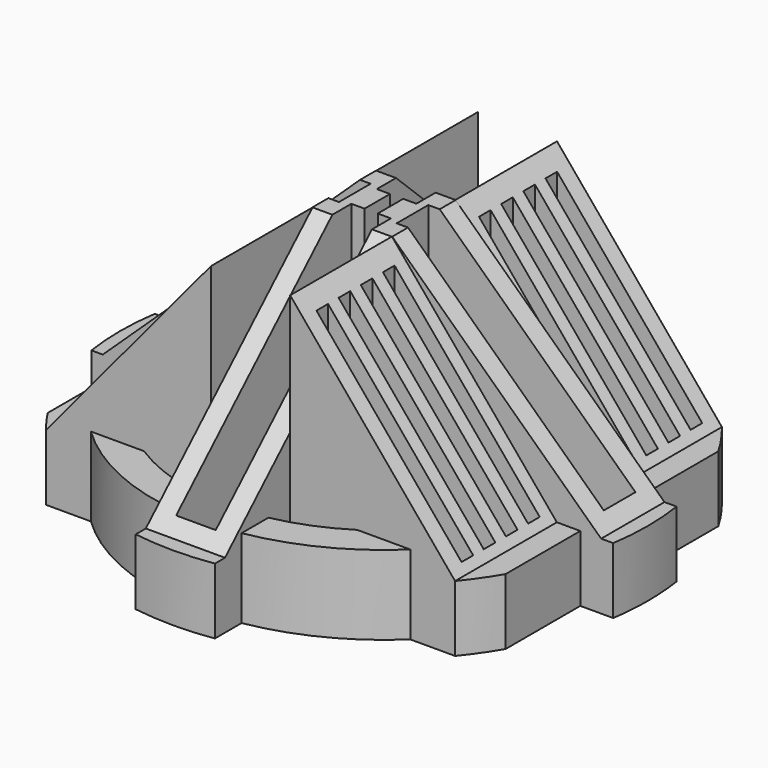
from build123d import *

# Parameters (mm, degrees)
F2_DEPTH  = 12.7
F3_DEPTH  = 25.4
F4_DEPTH  = 38.1
F5_DEPTH  = 50.8
F6_DEPTH  = 50.8
F7_DEPTH  = 50.8
F11_DEPTH = 15.24
F12_DEPTH = 15.24
F13_DEPTH = 15.24
F15_DEPTH = 15.24
F16_W     = 39.878
F16_H     = 7.62
F16_W_2   = 7.62
F16_H_2   = 42.164
F17_DEPTH = 46.99
F18_DEPTH = 50.8
F21_DEPTH = 24.4856
F19_W     = 27.94
F19_H     = 2.794
F22_DEPTH = 46.99
F24_DEPTH = 24.4856
F26_DEPTH = 24.4856
F28_DEPTH = 24.4856
F29_DEPTH = 50.801
F30_DEPTH = 25.4
F31_DEPTH = 10.16
F33_DEPTH = 25.4
F35_DEPTH = 46.99


# Not quite as in the source:
# - after a boolean that leaves OpenCascade's solid faulty, fix() repairs it
# - a feature names something its author has since deleted; it is built from what else it names


with BuildPart() as f2:
    # F1 (on Top) → F2 (new body)
    with BuildSketch(Plane.XY):
        with BuildLine():
            ThreePointArc((50.2252486305, -7.62), (50.6561083702, -3.8208225272), (50.8, 0))
            ThreePointArc((50.8, 0), (50.6561083702, 3.8208225272), (50.2252486305, 7.62))
            Line((50.2252486305, 7.62), (43.8856464383, 7.62))
            Line((43.8856464383, 7.62), (43.8856464383, -7.62))
            Line((43.8856464383, -7.62), (50.2252486305, -7.62))
        make_face()
        with BuildLine():
            Line((43.8856464383, 7.62), (50.2252486305, 7.62))
            ThreePointArc((50.2252486305, 7.62), (48.8754001329, 13.850460709), (46.7558464383, 19.8628))
            Line((46.7558464383, 19.8628), (43.8856464383, 19.8628))
            Line((43.8856464383, 19.8628), (43.8856464383, 7.62))
        make_face()
        with BuildLine():
            ThreePointArc((46.7558464383, -19.8628), (48.8754001329, -13.850460709), (50.2252486305, -7.62))
            Line((50.2252486305, -7.62), (43.8856464383, -7.62))
            Line((43.8856464383, -7.62), (43.8856464383, -19.8628))
            Line((43.8856464383, -19.8628), (46.7558464383, -19.8628))
        make_face()
        with BuildLine():
            Line((43.8856464383, 19.8628), (46.7558464383, 19.8628))
            ThreePointArc((46.7558464383, 19.8628), (43.4950311771, 26.2454236564), (39.3683940318, 32.1056))
            Line((39.3683940318, 32.1056), (30.7413882029, 32.1056))
            ThreePointArc((30.7413882029, 32.1056), (35.7808122406, 26.3730160468), (39.7652068542, 19.8628))
            Line((39.7652068542, 19.8628), (43.8856464383, 19.8628))
        make_face()
        with BuildLine():
            ThreePointArc((39.3683940318, -32.1056), (43.4950311771, -26.2454236564), (46.7558464383, -19.8628))
            Line((46.7558464383, -19.8628), (43.8856464383, -19.8628))
            Line((43.8856464383, -19.8628), (39.7652068542, -19.8628))
            ThreePointArc((39.7652068542, -19.8628), (35.7808122406, -26.3730160468), (30.7413882029, -32.1056))
            Line((30.7413882029, -32.1056), (39.3683940318, -32.1056))
        make_face()
        with BuildLine():
            Line((30.7413882029, 32.1056), (39.3683940318, 32.1056))
            ThreePointArc((39.3683940318, 32.1056), (25.1805025773, 44.1200894146), (7.62, 50.2252486305))
            Line((7.62, 50.2252486305), (7.62, 43.7919867099))
            ThreePointArc((7.62, 43.7919867099), (20.0509833873, 39.670651182), (30.7413882029, 32.1056))
        make_face()
        with BuildLine():
            ThreePointArc((7.62, -50.2252486305), (25.1805025773, -44.1200894146), (39.3683940318, -32.1056))
            Line((39.3683940318, -32.1056), (30.7413882029, -32.1056))
            ThreePointArc((30.7413882029, -32.1056), (20.0509833873, -39.670651182), (7.62, -43.7919867099))
            Line((7.62, -43.7919867099), (7.62, -50.2252486305))
        make_face()
        with BuildLine():
            Line((7.62, 43.7919867099), (7.62, 50.2252486305))
            ThreePointArc((7.62, 50.2252486305), (0, 50.8), (-7.62, 50.2252486305))
            Line((-7.62, 50.2252486305), (-7.62, 43.7919867099))
            ThreePointArc((-7.62, 43.7919867099), (0, 44.45), (7.62, 43.7919867099))
        make_face()
        with BuildLine():
            Line((20.5143961315, 32.1056), (30.7413882029, 32.1056))
            ThreePointArc((30.7413882029, 32.1056), (20.0509833873, 39.670651182), (7.62, 43.7919867099))
            Line((7.62, 43.7919867099), (7.62, 37.33022368))
            ThreePointArc((7.62, 37.33022368), (14.3076984372, 35.3114679025), (20.5143961315, 32.1056))
        make_face()
        with BuildLine():
            ThreePointArc((-7.62, -50.2252486305), (0, -50.8), (7.62, -50.2252486305))
            Line((7.62, -50.2252486305), (7.62, -43.7919867099))
            ThreePointArc((7.62, -43.7919867099), (0, -44.45), (-7.62, -43.7919867099))
            Line((-7.62, -43.7919867099), (-7.62, -50.2252486305))
        make_face()
        with BuildLine():
            ThreePointArc((7.62, -43.7919867099), (20.0509833873, -39.670651182), (30.7413882029, -32.1056))
            Line((30.7413882029, -32.1056), (20.5143961315, -32.1056))
            ThreePointArc((20.5143961315, -32.1056), (14.3076984372, -35.3114679025), (7.62, -37.33022368))
            Line((7.62, -37.33022368), (7.62, -43.7919867099))
        make_face()
        with BuildLine():
            Line((-7.62, 43.7919867099), (-7.62, 50.2252486305))
            ThreePointArc((-7.62, 50.2252486305), (-25.1805025773, 44.1200894146), (-39.3683940318, 32.1056))
            Line((-39.3683940318, 32.1056), (-30.7413882029, 32.1056))
            ThreePointArc((-30.7413882029, 32.1056), (-20.0509833873, 39.670651182), (-7.62, 43.7919867099))
        make_face()
        with BuildLine():
            ThreePointArc((-39.3683940318, -32.1056), (-25.1805025773, -44.1200894146), (-7.62, -50.2252486305))
            Line((-7.62, -50.2252486305), (-7.62, -43.7919867099))
            ThreePointArc((-7.62, -43.7919867099), (-20.0509833873, -39.670651182), (-30.7413882029, -32.1056))
            Line((-30.7413882029, -32.1056), (-39.3683940318, -32.1056))
        make_face()
        with BuildLine():
            Line((-30.7413882029, 32.1056), (-39.3683940318, 32.1056))
            ThreePointArc((-39.3683940318, 32.1056), (-43.4950311771, 26.2454236564), (-46.7558464383, 19.8628))
            Line((-46.7558464383, 19.8628), (-42.6407977939, 19.8628))
            Line((-42.6407977939, 19.8628), (-39.7652068542, 19.8628))
            ThreePointArc((-39.7652068542, 19.8628), (-35.7808122406, 26.3730160468), (-30.7413882029, 32.1056))
        make_face()
        with BuildLine():
            Line((-7.62, 37.33022368), (-7.62, 43.7919867099))
            ThreePointArc((-7.62, 43.7919867099), (-20.0509833873, 39.670651182), (-30.7413882029, 32.1056))
            Line((-30.7413882029, 32.1056), (-20.5143961315, 32.1056))
            ThreePointArc((-20.5143961315, 32.1056), (-14.3076984372, 35.3114679025), (-7.62, 37.33022368))
        make_face()
        with BuildLine():
            ThreePointArc((-46.7558464383, -19.8628), (-43.4950311771, -26.2454236564), (-39.3683940318, -32.1056))
            Line((-39.3683940318, -32.1056), (-30.7413882029, -32.1056))
            ThreePointArc((-30.7413882029, -32.1056), (-35.7808122406, -26.3730160468), (-39.7652068542, -19.8628))
            Line((-39.7652068542, -19.8628), (-42.6407977939, -19.8628))
            Line((-42.6407977939, -19.8628), (-46.7558464383, -19.8628))
        make_face()
        with BuildLine():
            ThreePointArc((-30.7413882029, -32.1056), (-20.0509833873, -39.670651182), (-7.62, -43.7919867099))
            Line((-7.62, -43.7919867099), (-7.62, -37.33022368))
            ThreePointArc((-7.62, -37.33022368), (-14.2009349705, -35.3545392554), (-20.32, -32.2289869527))
            ThreePointArc((-20.32, -32.2289869527), (-20.4172912734, -32.1674403249), (-20.5143961315, -32.1056))
            Line((-20.5143961315, -32.1056), (-30.7413882029, -32.1056))
        make_face()
        with BuildLine():
            Line((-42.6407977939, 19.8628), (-46.7558464383, 19.8628))
            ThreePointArc((-46.7558464383, 19.8628), (-48.8754001329, 13.850460709), (-50.2252486305, 7.62))
            Line((-50.2252486305, 7.62), (-42.6407977939, 7.62))
            Line((-42.6407977939, 7.62), (-42.6407977939, 19.8628))
        make_face()
        with BuildLine():
            ThreePointArc((-50.2252486305, -7.62), (-48.8754001329, -13.850460709), (-46.7558464383, -19.8628))
            Line((-46.7558464383, -19.8628), (-42.6407977939, -19.8628))
            Line((-42.6407977939, -19.8628), (-42.6407977939, -7.62))
            Line((-42.6407977939, -7.62), (-50.2252486305, -7.62))
        make_face()
        with BuildLine():
            Line((-42.6407977939, 7.62), (-50.2252486305, 7.62))
            ThreePointArc((-50.2252486305, 7.62), (-50.8, 0), (-50.2252486305, -7.62))
            Line((-50.2252486305, -7.62), (-42.6407977939, -7.62))
            Line((-42.6407977939, -7.62), (-42.6407977939, 7.62))
        make_face()
    extrude(amount=F2_DEPTH)

    # F1 (on Top) → F3 (join)
    with BuildSketch(Plane.XY):
        with BuildLine():
            ThreePointArc((-30.7413882029, -32.1056), (-20.0509833873, -39.670651182), (-7.62, -43.7919867099))
            Line((-7.62, -43.7919867099), (-7.62, -37.33022368))
            ThreePointArc((-7.62, -37.33022368), (-14.2009349705, -35.3545392554), (-20.32, -32.2289869527))
            ThreePointArc((-20.32, -32.2289869527), (-20.4172912734, -32.1674403249), (-20.5143961315, -32.1056))
            Line((-20.5143961315, -32.1056), (-30.7413882029, -32.1056))
        make_face()
        with BuildLine():
            ThreePointArc((7.62, -43.7919867099), (20.0509833873, -39.670651182), (30.7413882029, -32.1056))
            Line((30.7413882029, -32.1056), (20.5143961315, -32.1056))
            ThreePointArc((20.5143961315, -32.1056), (14.3076984372, -35.3114679025), (7.62, -37.33022368))
            Line((7.62, -37.33022368), (7.62, -43.7919867099))
        make_face()
        with BuildLine():
            Line((20.5143961315, -32.1056), (30.7413882029, -32.1056))
            ThreePointArc((30.7413882029, -32.1056), (35.7808122406, -26.3730160468), (39.7652068542, -19.8628))
            Line((39.7652068542, -19.8628), (32.5127540538, -19.8628))
            ThreePointArc((32.5127540538, -19.8628), (27.2110492659, -26.667748271), (20.5143961315, -32.1056))
        make_face()
        with BuildLine():
            Line((7.62, 37.33022368), (7.62, 43.7919867099))
            ThreePointArc((7.62, 43.7919867099), (0, 44.45), (-7.62, 43.7919867099))
            Line((-7.62, 43.7919867099), (-7.62, 37.33022368))
            ThreePointArc((-7.62, 37.33022368), (0, 38.1), (7.62, 37.33022368))
        make_face()
        with BuildLine():
            ThreePointArc((-7.62, -43.7919867099), (0, -44.45), (7.62, -43.7919867099))
            Line((7.62, -43.7919867099), (7.62, -37.33022368))
            ThreePointArc((7.62, -37.33022368), (0, -38.1), (-7.62, -37.33022368))
            Line((-7.62, -37.33022368), (-7.62, -43.7919867099))
        make_face()
        with BuildLine():
            Line((-37.33022368, 7.62), (-42.6407977939, 7.62))
            Line((-42.6407977939, 7.62), (-42.6407977939, -7.62))
            Line((-42.6407977939, -7.62), (-37.33022368, -7.62))
            ThreePointArc((-37.33022368, -7.62), (-38.1, 0), (-37.33022368, 7.62))
        make_face()
        with BuildLine():
            Line((-42.6407977939, -7.62), (-42.6407977939, -19.8628))
            Line((-42.6407977939, -19.8628), (-39.7652068542, -19.8628))
            Line((-39.7652068542, -19.8628), (-32.5127540538, -19.8628))
            ThreePointArc((-32.5127540538, -19.8628), (-35.4539408619, -13.9509167211), (-37.33022368, -7.62))
            Line((-37.33022368, -7.62), (-42.6407977939, -7.62))
        make_face()
        with BuildLine():
            ThreePointArc((-39.7652068542, -19.8628), (-35.7808122406, -26.3730160468), (-30.7413882029, -32.1056))
            Line((-30.7413882029, -32.1056), (-20.5143961315, -32.1056))
            ThreePointArc((-20.5143961315, -32.1056), (-27.2110492659, -26.667748271), (-32.5127540538, -19.8628))
            Line((-32.5127540538, -19.8628), (-39.7652068542, -19.8628))
        make_face()
        with BuildLine():
            Line((-39.7652068542, 19.8628), (-42.6407977939, 19.8628))
            Line((-42.6407977939, 19.8628), (-42.6407977939, 7.62))
            Line((-42.6407977939, 7.62), (-37.33022368, 7.62))
            ThreePointArc((-37.33022368, 7.62), (-35.4539408619, 13.9509167211), (-32.5127540538, 19.8628))
            Line((-32.5127540538, 19.8628), (-39.7652068542, 19.8628))
        make_face()
        with BuildLine():
            Line((-20.5143961315, 32.1056), (-30.7413882029, 32.1056))
            ThreePointArc((-30.7413882029, 32.1056), (-35.7808122406, 26.3730160468), (-39.7652068542, 19.8628))
            Line((-39.7652068542, 19.8628), (-32.5127540538, 19.8628))
            ThreePointArc((-32.5127540538, 19.8628), (-27.2110492659, 26.667748271), (-20.5143961315, 32.1056))
        make_face()
        with BuildLine():
            Line((-7.62, 37.33022368), (-7.62, 43.7919867099))
            ThreePointArc((-7.62, 43.7919867099), (-20.0509833873, 39.670651182), (-30.7413882029, 32.1056))
            Line((-30.7413882029, 32.1056), (-20.5143961315, 32.1056))
            ThreePointArc((-20.5143961315, 32.1056), (-14.3076984372, 35.3114679025), (-7.62, 37.33022368))
        make_face()
        with BuildLine():
            ThreePointArc((39.7652068542, 19.8628), (35.7808122406, 26.3730160468), (30.7413882029, 32.1056))
            Line((30.7413882029, 32.1056), (20.5143961315, 32.1056))
            ThreePointArc((20.5143961315, 32.1056), (27.2110492659, 26.667748271), (32.5127540538, 19.8628))
            Line((32.5127540538, 19.8628), (39.7652068542, 19.8628))
        make_face()
        with BuildLine():
            Line((37.33022368, 7.62), (43.8856464383, 7.62))
            Line((43.8856464383, 7.62), (43.8856464383, 19.8628))
            Line((43.8856464383, 19.8628), (39.7652068542, 19.8628))
            Line((39.7652068542, 19.8628), (32.5127540538, 19.8628))
            ThreePointArc((32.5127540538, 19.8628), (35.4539408619, 13.9509167211), (37.33022368, 7.62))
        make_face()
        with BuildLine():
            Line((43.8856464383, -19.8628), (43.8856464383, -7.62))
            Line((43.8856464383, -7.62), (37.33022368, -7.62))
            ThreePointArc((37.33022368, -7.62), (35.4539408619, -13.9509167211), (32.5127540538, -19.8628))
            Line((32.5127540538, -19.8628), (39.7652068542, -19.8628))
            Line((39.7652068542, -19.8628), (43.8856464383, -19.8628))
        make_face()
        with BuildLine():
            Line((43.8856464383, -7.62), (43.8856464383, 7.62))
            Line((43.8856464383, 7.62), (37.33022368, 7.62))
            ThreePointArc((37.33022368, 7.62), (38.1, 0), (37.33022368, -7.62))
            Line((37.33022368, -7.62), (43.8856464383, -7.62))
        make_face()
        with BuildLine():
            Line((20.5143961315, 32.1056), (30.7413882029, 32.1056))
            ThreePointArc((30.7413882029, 32.1056), (20.0509833873, 39.670651182), (7.62, 43.7919867099))
            Line((7.62, 43.7919867099), (7.62, 37.33022368))
            ThreePointArc((7.62, 37.33022368), (14.3076984372, 35.3114679025), (20.5143961315, 32.1056))
        make_face()
    extrude(amount=F3_DEPTH)

    # F1 (on Top) → F4 (join)
    with BuildSketch(Plane.XY):
        with BuildLine():
            ThreePointArc((-7.62, -37.33022368), (0, -38.1), (7.62, -37.33022368))
            Line((7.62, -37.33022368), (7.62, -32.1056))
            Line((7.62, -32.1056), (7.62, -30.8220391928))
            ThreePointArc((7.62, -30.8220391928), (0, -31.75), (-7.62, -30.8220391928))
            Line((-7.62, -30.8220391928), (-7.62, -32.1056))
            Line((-7.62, -32.1056), (-7.62, -37.33022368))
        make_face()
        with BuildLine():
            Line((-7.62, 32.1056), (-7.62, 37.33022368))
            ThreePointArc((-7.62, 37.33022368), (-14.3076984372, 35.3114679025), (-20.5143961315, 32.1056))
            Line((-20.5143961315, 32.1056), (-7.62, 32.1056))
        make_face()
        with BuildLine():
            ThreePointArc((-24.769571578, 19.8628), (-17.0967048776, 26.7537881865), (-7.62, 30.8220391928))
            Line((-7.62, 30.8220391928), (-7.62, 32.1056))
            Line((-7.62, 32.1056), (-20.5143961315, 32.1056))
            ThreePointArc((-20.5143961315, 32.1056), (-27.2110492659, 26.667748271), (-32.5127540538, 19.8628))
            Line((-32.5127540538, 19.8628), (-24.769571578, 19.8628))
        make_face()
        with BuildLine():
            ThreePointArc((-30.8220391928, 7.62), (-28.4618751136, 14.0706845966), (-24.769571578, 19.8628))
            Line((-24.769571578, 19.8628), (-32.5127540538, 19.8628))
            ThreePointArc((-32.5127540538, 19.8628), (-35.4539408619, 13.9509167211), (-37.33022368, 7.62))
            Line((-37.33022368, 7.62), (-30.8220391928, 7.62))
        make_face()
        with BuildLine():
            ThreePointArc((-30.8220391928, -7.62), (-31.75, 0), (-30.8220391928, 7.62))
            Line((-30.8220391928, 7.62), (-37.33022368, 7.62))
            ThreePointArc((-37.33022368, 7.62), (-38.1, 0), (-37.33022368, -7.62))
            Line((-37.33022368, -7.62), (-30.8220391928, -7.62))
        make_face()
        with BuildLine():
            Line((-32.5127540538, -19.8628), (-24.769571578, -19.8628))
            ThreePointArc((-24.769571578, -19.8628), (-28.4618751136, -14.0706845966), (-30.8220391928, -7.62))
            Line((-30.8220391928, -7.62), (-37.33022368, -7.62))
            ThreePointArc((-37.33022368, -7.62), (-35.4539408619, -13.9509167211), (-32.5127540538, -19.8628))
        make_face()
        with BuildLine():
            Line((-7.62, -32.1056), (-7.62, -30.8220391928))
            ThreePointArc((-7.62, -30.8220391928), (-17.0967048776, -26.7537881865), (-24.769571578, -19.8628))
            Line((-24.769571578, -19.8628), (-32.5127540538, -19.8628))
            ThreePointArc((-32.5127540538, -19.8628), (-27.2110492659, -26.667748271), (-20.5143961315, -32.1056))
            Line((-20.5143961315, -32.1056), (-20.32, -32.1056))
            Line((-20.32, -32.1056), (-7.62, -32.1056))
        make_face()
        with BuildLine():
            Line((-20.32, -32.1056), (-20.5143961315, -32.1056))
            ThreePointArc((-20.5143961315, -32.1056), (-20.4172912734, -32.1674403249), (-20.32, -32.2289869527))
            Line((-20.32, -32.2289869527), (-20.32, -32.1056))
        make_face()
        with BuildLine():
            ThreePointArc((-20.32, -32.2289869527), (-14.2009349705, -35.3545392554), (-7.62, -37.33022368))
            Line((-7.62, -37.33022368), (-7.62, -32.1056))
            Line((-7.62, -32.1056), (-20.32, -32.1056))
            Line((-20.32, -32.1056), (-20.32, -32.2289869527))
        make_face()
        with BuildLine():
            ThreePointArc((7.62, -37.33022368), (14.3076984372, -35.3114679025), (20.5143961315, -32.1056))
            Line((20.5143961315, -32.1056), (7.62, -32.1056))
            Line((7.62, -32.1056), (7.62, -37.33022368))
        make_face()
        with BuildLine():
            ThreePointArc((20.5143961315, -32.1056), (27.2110492659, -26.667748271), (32.5127540538, -19.8628))
            Line((32.5127540538, -19.8628), (24.769571578, -19.8628))
            ThreePointArc((24.769571578, -19.8628), (17.0967048776, -26.7537881865), (7.62, -30.8220391928))
            Line((7.62, -30.8220391928), (7.62, -32.1056))
            Line((7.62, -32.1056), (20.5143961315, -32.1056))
        make_face()
        with BuildLine():
            ThreePointArc((32.5127540538, -19.8628), (35.4539408619, -13.9509167211), (37.33022368, -7.62))
            Line((37.33022368, -7.62), (30.8220391928, -7.62))
            ThreePointArc((30.8220391928, -7.62), (28.4618751136, -14.0706845966), (24.769571578, -19.8628))
            Line((24.769571578, -19.8628), (32.5127540538, -19.8628))
        make_face()
        with BuildLine():
            ThreePointArc((37.33022368, -7.62), (38.1, 0), (37.33022368, 7.62))
            Line((37.33022368, 7.62), (30.8220391928, 7.62))
            ThreePointArc((30.8220391928, 7.62), (31.5171559977, 3.8381477062), (31.75, 0))
            ThreePointArc((31.75, 0), (31.5171559977, -3.8381477062), (30.8220391928, -7.62))
            Line((30.8220391928, -7.62), (37.33022368, -7.62))
        make_face()
        with BuildLine():
            Line((30.8220391928, 7.62), (37.33022368, 7.62))
            ThreePointArc((37.33022368, 7.62), (35.4539408619, 13.9509167211), (32.5127540538, 19.8628))
            Line((32.5127540538, 19.8628), (24.769571578, 19.8628))
            ThreePointArc((24.769571578, 19.8628), (28.4618751136, 14.0706845966), (30.8220391928, 7.62))
        make_face()
        with BuildLine():
            Line((24.769571578, 19.8628), (32.5127540538, 19.8628))
            ThreePointArc((32.5127540538, 19.8628), (27.2110492659, 26.667748271), (20.5143961315, 32.1056))
            Line((20.5143961315, 32.1056), (7.62, 32.1056))
            Line((7.62, 32.1056), (7.62, 30.8220391928))
            ThreePointArc((7.62, 30.8220391928), (17.0967048776, 26.7537881865), (24.769571578, 19.8628))
        make_face()
        with BuildLine():
            Line((7.62, 32.1056), (20.5143961315, 32.1056))
            ThreePointArc((20.5143961315, 32.1056), (14.3076984372, 35.3114679025), (7.62, 37.33022368))
            Line((7.62, 37.33022368), (7.62, 32.1056))
        make_face()
        with BuildLine():
            Line((7.62, 32.1056), (7.62, 37.33022368))
            ThreePointArc((7.62, 37.33022368), (0, 38.1), (-7.62, 37.33022368))
            Line((-7.62, 37.33022368), (-7.62, 32.1056))
            Line((-7.62, 32.1056), (-7.62, 30.8220391928))
            ThreePointArc((-7.62, 30.8220391928), (0, 31.75), (7.62, 30.8220391928))
            Line((7.62, 30.8220391928), (7.62, 32.1056))
        make_face()
    extrude(amount=F4_DEPTH)

    # F1 (on Top) → F5 (join)
    with BuildSketch(Plane.XY):
        with BuildLine():
            Line((7.62, 24.230055716), (7.62, 30.8220391928))
            ThreePointArc((7.62, 30.8220391928), (0, 31.75), (-7.62, 30.8220391928))
            Line((-7.62, 30.8220391928), (-7.62, 24.230055716))
            ThreePointArc((-7.62, 24.230055716), (0, 25.4), (7.62, 24.230055716))
        make_face()
        with BuildLine():
            ThreePointArc((-7.62, -30.8220391928), (0, -31.75), (7.62, -30.8220391928))
            Line((7.62, -30.8220391928), (7.62, -24.230055716))
            ThreePointArc((7.62, -24.230055716), (0, -25.4), (-7.62, -24.230055716))
            Line((-7.62, -24.230055716), (-7.62, -30.8220391928))
        make_face()
        with BuildLine():
            ThreePointArc((7.62, -30.8220391928), (17.0967048776, -26.7537881865), (24.769571578, -19.8628))
            Line((24.769571578, -19.8628), (15.8312720954, -19.8628))
            ThreePointArc((15.8312720954, -19.8628), (11.9272281502, -22.4254593856), (7.62, -24.230055716))
            Line((7.62, -24.230055716), (7.62, -30.8220391928))
        make_face()
        with BuildLine():
            Line((15.8312720954, 19.8628), (24.769571578, 19.8628))
            ThreePointArc((24.769571578, 19.8628), (17.0967048776, 26.7537881865), (7.62, 30.8220391928))
            Line((7.62, 30.8220391928), (7.62, 24.230055716))
            ThreePointArc((7.62, 24.230055716), (11.9272281502, 22.4254593856), (15.8312720954, 19.8628))
        make_face()
        with BuildLine():
            Line((-24.230055716, 7.62), (-30.8220391928, 7.62))
            ThreePointArc((-30.8220391928, 7.62), (-31.75, 0), (-30.8220391928, -7.62))
            Line((-30.8220391928, -7.62), (-24.230055716, -7.62))
            ThreePointArc((-24.230055716, -7.62), (-25.4, 0), (-24.230055716, 7.62))
        make_face()
        with BuildLine():
            Line((-7.62, 24.230055716), (-7.62, 30.8220391928))
            ThreePointArc((-7.62, 30.8220391928), (-17.0967048776, 26.7537881865), (-24.769571578, 19.8628))
            Line((-24.769571578, 19.8628), (-15.8312720954, 19.8628))
            ThreePointArc((-15.8312720954, 19.8628), (-11.9272281502, 22.4254593856), (-7.62, 24.230055716))
        make_face()
        with BuildLine():
            ThreePointArc((31.75, 0), (31.5171559977, 3.8381477062), (30.8220391928, 7.62))
            Line((30.8220391928, 7.62), (24.230055716, 7.62))
            ThreePointArc((24.230055716, 7.62), (25.1058102357, 3.8546455618), (25.4, 0))
            ThreePointArc((25.4, 0), (25.1058102357, -3.8546455618), (24.230055716, -7.62))
            Line((24.230055716, -7.62), (30.8220391928, -7.62))
            ThreePointArc((30.8220391928, -7.62), (31.5171559977, -3.8381477062), (31.75, 0))
        make_face()
        with BuildLine():
            ThreePointArc((-24.769571578, -19.8628), (-17.0967048776, -26.7537881865), (-7.62, -30.8220391928))
            Line((-7.62, -30.8220391928), (-7.62, -24.230055716))
            ThreePointArc((-7.62, -24.230055716), (-11.9272281502, -22.4254593856), (-15.8312720954, -19.8628))
            Line((-15.8312720954, -19.8628), (-20.32, -19.8628))
            Line((-20.32, -19.8628), (-24.769571578, -19.8628))
        make_face()
        with BuildLine():
            ThreePointArc((-30.8220391928, -7.62), (-28.4618751136, -14.0706845966), (-24.769571578, -19.8628))
            Line((-24.769571578, -19.8628), (-20.32, -19.8628))
            Line((-20.32, -19.8628), (-15.8312720954, -19.8628))
            ThreePointArc((-15.8312720954, -19.8628), (-20.9451434577, -14.3687496163), (-24.230055716, -7.62))
            Line((-24.230055716, -7.62), (-30.8220391928, -7.62))
        make_face()
    extrude(amount=F5_DEPTH)



with BuildPart() as f2b:
    # F1 (on Top) → F2, piece 2 (new body)
    with BuildSketch(Plane.XY):
        Polygon((7.62, 2.54), (7.62, 7.62), (2.54, 7.62), align=None)
    extrude(amount=F2_DEPTH)


with BuildPart() as f2c:
    # F1 (on Top) → F2, piece 3 (new body)
    with BuildSketch(Plane.XY):
        Polygon((2.54, -7.62), (7.62, -7.62), (7.62, -2.54), align=None)
    extrude(amount=F2_DEPTH)


with BuildPart() as f2d:
    # F1 (on Top) → F2, piece 4 (new body)
    with BuildSketch(Plane.XY):
        Polygon((-7.62, 2.54), (-2.54, 7.62), (-7.62, 7.62), align=None)
    extrude(amount=F2_DEPTH)


with BuildPart() as f2_1:
    add(f2.part)

    add(f2b.part)  # F6 merges F2b

    add(f2c.part)  # F6 merges F2c

    add(f2d.part)  # F6 merges F2d
    # F1 (on Top) → F6 (join)
    with BuildSketch(Plane.XY):
        with BuildLine():
            ThreePointArc((-7.62, -50.2252486305), (0, -50.8), (7.62, -50.2252486305))
            Line((7.62, -50.2252486305), (7.62, -43.7919867099))
            ThreePointArc((7.62, -43.7919867099), (0, -44.45), (-7.62, -43.7919867099))
            Line((-7.62, -43.7919867099), (-7.62, -50.2252486305))
        make_face()
        with BuildLine():
            ThreePointArc((-7.62, -37.33022368), (0, -38.1), (7.62, -37.33022368))
            Line((7.62, -37.33022368), (7.62, -32.1056))
            Line((7.62, -32.1056), (7.62, -30.8220391928))
            ThreePointArc((7.62, -30.8220391928), (0, -31.75), (-7.62, -30.8220391928))
            Line((-7.62, -30.8220391928), (-7.62, -32.1056))
            Line((-7.62, -32.1056), (-7.62, -37.33022368))
        make_face()
        with BuildLine():
            ThreePointArc((-7.62, -30.8220391928), (0, -31.75), (7.62, -30.8220391928))
            Line((7.62, -30.8220391928), (7.62, -24.230055716))
            ThreePointArc((7.62, -24.230055716), (0, -25.4), (-7.62, -24.230055716))
            Line((-7.62, -24.230055716), (-7.62, -30.8220391928))
        make_face()
        with BuildLine():
            ThreePointArc((-7.62, -43.7919867099), (0, -44.45), (7.62, -43.7919867099))
            Line((7.62, -43.7919867099), (7.62, -37.33022368))
            ThreePointArc((7.62, -37.33022368), (0, -38.1), (-7.62, -37.33022368))
            Line((-7.62, -37.33022368), (-7.62, -43.7919867099))
        make_face()
        with BuildLine():
            ThreePointArc((-7.62, -24.230055716), (0, -25.4), (7.62, -24.230055716))
            Line((7.62, -24.230055716), (7.62, -19.8628))
            Line((7.62, -19.8628), (7.62, -17.78))
            Line((7.62, -17.78), (0, -10.16))
            Line((0, -10.16), (-7.62, -17.78))
            Line((-7.62, -17.78), (-7.62, -19.8628))
            Line((-7.62, -19.8628), (-7.62, -24.230055716))
        make_face()
        with BuildLine():
            Line((7.62, 19.8628), (7.62, 24.230055716))
            ThreePointArc((7.62, 24.230055716), (0, 25.4), (-7.62, 24.230055716))
            Line((-7.62, 24.230055716), (-7.62, 19.8628))
            Line((-7.62, 19.8628), (-7.62, 17.78))
            Line((-7.62, 17.78), (0, 10.16))
            Line((0, 10.16), (7.62, 17.78))
            Line((7.62, 17.78), (7.62, 19.8628))
        make_face()
        with BuildLine():
            Line((7.62, 24.230055716), (7.62, 30.8220391928))
            ThreePointArc((7.62, 30.8220391928), (0, 31.75), (-7.62, 30.8220391928))
            Line((-7.62, 30.8220391928), (-7.62, 24.230055716))
            ThreePointArc((-7.62, 24.230055716), (0, 25.4), (7.62, 24.230055716))
        make_face()
        with BuildLine():
            Line((7.62, 32.1056), (7.62, 37.33022368))
            ThreePointArc((7.62, 37.33022368), (0, 38.1), (-7.62, 37.33022368))
            Line((-7.62, 37.33022368), (-7.62, 32.1056))
            Line((-7.62, 32.1056), (-7.62, 30.8220391928))
            ThreePointArc((-7.62, 30.8220391928), (0, 31.75), (7.62, 30.8220391928))
            Line((7.62, 30.8220391928), (7.62, 32.1056))
        make_face()
        with BuildLine():
            Line((7.62, 37.33022368), (7.62, 43.7919867099))
            ThreePointArc((7.62, 43.7919867099), (0, 44.45), (-7.62, 43.7919867099))
            Line((-7.62, 43.7919867099), (-7.62, 37.33022368))
            ThreePointArc((-7.62, 37.33022368), (0, 38.1), (7.62, 37.33022368))
        make_face()
        with BuildLine():
            Line((7.62, 43.7919867099), (7.62, 50.2252486305))
            ThreePointArc((7.62, 50.2252486305), (0, 50.8), (-7.62, 50.2252486305))
            Line((-7.62, 50.2252486305), (-7.62, 43.7919867099))
            ThreePointArc((-7.62, 43.7919867099), (0, 44.45), (7.62, 43.7919867099))
        make_face()
        Polygon((7.62, -17.78), (7.62, -7.62), (2.54, -7.62), (0, -10.16), align=None)
        Polygon((-2.54, 7.62), (0, 10.16), (-7.62, 17.78), (-7.62, 7.62), align=None)
        Polygon((-7.62, -7.62), (-2.54, -7.62), (-7.62, -2.54), align=None)
        Polygon((-7.62, -17.78), (0, -10.16), (-2.54, -7.62), (-7.62, -7.62), align=None)
        Polygon((7.62, -2.54), (7.62, 2.54), (2.54, 7.62), (0, 7.62), (-2.54, 7.62), (-7.62, 2.54), (-7.62, -2.54), (-2.54, -7.62), (0, -7.62), (2.54, -7.62), align=None)
        Polygon((2.54, 7.62), (7.62, 7.62), (7.62, 17.78), (0, 10.16), align=None)
        Polygon((0, 7.62), (2.54, 7.62), (0, 10.16), (-2.54, 7.62), align=None)
        Polygon((0, -10.16), (2.54, -7.62), (0, -7.62), (-2.54, -7.62), align=None)
        Polygon((-7.62, 2.54), (-2.54, 7.62), (-7.62, 7.62), align=None)
        Polygon((2.54, -7.62), (7.62, -7.62), (7.62, -2.54), align=None)
        Polygon((7.62, 2.54), (7.62, 7.62), (2.54, 7.62), align=None)
    extrude(amount=F6_DEPTH)

    # F1 (on Top) → F7 (join)
    with BuildSketch(Plane.XY):
        with BuildLine():
            ThreePointArc((-24.230055716, -7.62), (-20.9451434577, -14.3687496163), (-15.8312720954, -19.8628))
            Line((-15.8312720954, -19.8628), (-7.62, -19.8628))
            Line((-7.62, -19.8628), (-7.62, -17.78))
            Line((-7.62, -17.78), (-7.62, -7.62))
            Line((-7.62, -7.62), (-17.78, -7.62))
            Line((-17.78, -7.62), (-24.230055716, -7.62))
        make_face()
        with BuildLine():
            ThreePointArc((-15.8312720954, -19.8628), (-11.9272281502, -22.4254593856), (-7.62, -24.230055716))
            Line((-7.62, -24.230055716), (-7.62, -19.8628))
            Line((-7.62, -19.8628), (-15.8312720954, -19.8628))
        make_face()
        with BuildLine():
            Line((-42.6407977939, 7.62), (-50.2252486305, 7.62))
            ThreePointArc((-50.2252486305, 7.62), (-50.8, 0), (-50.2252486305, -7.62))
            Line((-50.2252486305, -7.62), (-42.6407977939, -7.62))
            Line((-42.6407977939, -7.62), (-42.6407977939, 7.62))
        make_face()
        with BuildLine():
            Line((-37.33022368, 7.62), (-42.6407977939, 7.62))
            Line((-42.6407977939, 7.62), (-42.6407977939, -7.62))
            Line((-42.6407977939, -7.62), (-37.33022368, -7.62))
            ThreePointArc((-37.33022368, -7.62), (-38.1, 0), (-37.33022368, 7.62))
        make_face()
        with BuildLine():
            ThreePointArc((-30.8220391928, -7.62), (-31.75, 0), (-30.8220391928, 7.62))
            Line((-30.8220391928, 7.62), (-37.33022368, 7.62))
            ThreePointArc((-37.33022368, 7.62), (-38.1, 0), (-37.33022368, -7.62))
            Line((-37.33022368, -7.62), (-30.8220391928, -7.62))
        make_face()
        with BuildLine():
            Line((-24.230055716, 7.62), (-30.8220391928, 7.62))
            ThreePointArc((-30.8220391928, 7.62), (-31.75, 0), (-30.8220391928, -7.62))
            Line((-30.8220391928, -7.62), (-24.230055716, -7.62))
            ThreePointArc((-24.230055716, -7.62), (-25.4, 0), (-24.230055716, 7.62))
        make_face()
        with BuildLine():
            Line((-17.78, 7.62), (-24.230055716, 7.62))
            ThreePointArc((-24.230055716, 7.62), (-25.4, 0), (-24.230055716, -7.62))
            Line((-24.230055716, -7.62), (-17.78, -7.62))
            Line((-17.78, -7.62), (-10.16, 0))
            Line((-10.16, 0), (-17.78, 7.62))
        make_face()
        Polygon((-7.62, -7.62), (-2.54, -7.62), (-7.62, -2.54), align=None)
        with BuildLine():
            ThreePointArc((25.4, 0), (25.1058102357, 3.8546455618), (24.230055716, 7.62))
            Line((24.230055716, 7.62), (17.78, 7.62))
            Line((17.78, 7.62), (10.16, 0))
            Line((10.16, 0), (17.78, -7.62))
            Line((17.78, -7.62), (24.230055716, -7.62))
            ThreePointArc((24.230055716, -7.62), (25.1058102357, -3.8546455618), (25.4, 0))
        make_face()
        with BuildLine():
            ThreePointArc((31.75, 0), (31.5171559977, 3.8381477062), (30.8220391928, 7.62))
            Line((30.8220391928, 7.62), (24.230055716, 7.62))
            ThreePointArc((24.230055716, 7.62), (25.1058102357, 3.8546455618), (25.4, 0))
            ThreePointArc((25.4, 0), (25.1058102357, -3.8546455618), (24.230055716, -7.62))
            Line((24.230055716, -7.62), (30.8220391928, -7.62))
            ThreePointArc((30.8220391928, -7.62), (31.5171559977, -3.8381477062), (31.75, 0))
        make_face()
        with BuildLine():
            ThreePointArc((37.33022368, -7.62), (38.1, 0), (37.33022368, 7.62))
            Line((37.33022368, 7.62), (30.8220391928, 7.62))
            ThreePointArc((30.8220391928, 7.62), (31.5171559977, 3.8381477062), (31.75, 0))
            ThreePointArc((31.75, 0), (31.5171559977, -3.8381477062), (30.8220391928, -7.62))
            Line((30.8220391928, -7.62), (37.33022368, -7.62))
        make_face()
        with BuildLine():
            ThreePointArc((50.2252486305, -7.62), (50.6561083702, -3.8208225272), (50.8, 0))
            ThreePointArc((50.8, 0), (50.6561083702, 3.8208225272), (50.2252486305, 7.62))
            Line((50.2252486305, 7.62), (43.8856464383, 7.62))
            Line((43.8856464383, 7.62), (43.8856464383, -7.62))
            Line((43.8856464383, -7.62), (50.2252486305, -7.62))
        make_face()
        Polygon((-10.16, 0), (-17.78, -7.62), (-7.62, -7.62), (-7.62, -2.54), align=None)
        Polygon((10.16, 0), (17.78, 7.62), (7.62, 7.62), (7.62, 2.54), align=None)
        Polygon((-7.62, -2.54), (-7.62, 2.54), (-10.16, 0), align=None)
        Polygon((7.62, -2.54), (10.16, 0), (7.62, 2.54), align=None)
        Polygon((-7.62, 7.62), (-17.78, 7.62), (-10.16, 0), (-7.62, 2.54), align=None)
        Polygon((7.62, -7.62), (17.78, -7.62), (10.16, 0), (7.62, -2.54), align=None)
        with BuildLine():
            ThreePointArc((15.8312720954, -19.8628), (20.9451434577, -14.3687496163), (24.230055716, -7.62))
            Line((24.230055716, -7.62), (17.78, -7.62))
            Line((17.78, -7.62), (7.62, -7.62))
            Line((7.62, -7.62), (7.62, -17.78))
            Line((7.62, -17.78), (7.62, -19.8628))
            Line((7.62, -19.8628), (15.8312720954, -19.8628))
        make_face()
        with BuildLine():
            Line((17.78, 7.62), (24.230055716, 7.62))
            ThreePointArc((24.230055716, 7.62), (20.9451434577, 14.3687496163), (15.8312720954, 19.8628))
            Line((15.8312720954, 19.8628), (7.62, 19.8628))
            Line((7.62, 19.8628), (7.62, 17.78))
            Line((7.62, 17.78), (7.62, 7.62))
            Line((7.62, 7.62), (17.78, 7.62))
        make_face()
        with BuildLine():
            Line((-7.62, 19.8628), (-15.8312720954, 19.8628))
            ThreePointArc((-15.8312720954, 19.8628), (-20.9451434577, 14.3687496163), (-24.230055716, 7.62))
            Line((-24.230055716, 7.62), (-17.78, 7.62))
            Line((-17.78, 7.62), (-7.62, 7.62))
            Line((-7.62, 7.62), (-7.62, 17.78))
            Line((-7.62, 17.78), (-7.62, 19.8628))
        make_face()
        with BuildLine():
            Line((43.8856464383, -7.62), (43.8856464383, 7.62))
            Line((43.8856464383, 7.62), (37.33022368, 7.62))
            ThreePointArc((37.33022368, 7.62), (38.1, 0), (37.33022368, -7.62))
            Line((37.33022368, -7.62), (43.8856464383, -7.62))
        make_face()
    extrude(amount=F7_DEPTH)

    # F8 (on face) → F11 (cut)
    with BuildSketch(Plane.XZ.offset(7.62)):
        Polygon((-55.5124618113, 12.7), (-48.0377227068, 12.7), (-7.6606776565, 50.8), (-7.6606776565, 65.3503203437), (-55.9246055782, 65.3503203437), align=None)
    extrude(amount=-F11_DEPTH, mode=Mode.SUBTRACT)

    # F9 (on face) → F12 (cut)
    with BuildSketch(Plane.XZ.offset(7.62)):
        Polygon((7.6703908853, 50.8), (47.8966571391, 12.7), (55.3924329579, 12.7), (55.3924329579, 55.8396019042), (7.6703908853, 53.9275594056), align=None)
    extrude(amount=-F12_DEPTH, mode=Mode.SUBTRACT)

    # F10 (on face) → F13 (cut)
    with BuildSketch(Plane.YZ.offset(7.62)):
        Polygon((-58.5949867964, 12.7), (-47.7943047881, 12.7), (-7.6625170186, 50.8), (-7.6625170186, 52.6358112693), (-57.5197674334, 52.6358112693), align=None)
    extrude(amount=-F13_DEPTH, mode=Mode.SUBTRACT)

    # F14 (on face) → F15 (cut)
    with BuildSketch(Plane(origin=(-7.62, 0, 0), x_dir=(0, -1, 0), z_dir=(-1, 0, 0))):
        Polygon((-54.0386848152, 12.7), (-47.7350726724, 12.7), (-7.6549332589, 50.8), (-7.6549332589, 52.5853484869), (-58.2393705845, 53.2422102988), align=None)
    extrude(amount=-F15_DEPTH, mode=Mode.SUBTRACT)

    # F16 (on offset) → F17 (cut)
    with BuildSketch(Plane.XY.offset(50.8)):
        with Locations((25.4176571391, 0)):
            Rectangle(F16_W, F16_H)
        with Locations((-25.5587227068, 0)):
            Rectangle(F16_W, F16_H)
        with Locations((0, 24.1130726724)):
            Rectangle(F16_W_2, F16_H_2)
        with Locations((0, -24.1723047881)):
            Rectangle(F16_W_2, F16_H_2)
    extrude(amount=-F17_DEPTH, mode=Mode.SUBTRACT)

    # F1 (on Top) → F18 (join)
    with BuildSketch(Plane.XY):
        with BuildLine():
            ThreePointArc((-24.230055716, -7.62), (-20.9451434577, -14.3687496163), (-15.8312720954, -19.8628))
            Line((-15.8312720954, -19.8628), (-7.62, -19.8628))
            Line((-7.62, -19.8628), (-7.62, -17.78))
            Line((-7.62, -17.78), (-7.62, -7.62))
            Line((-7.62, -7.62), (-17.78, -7.62))
            Line((-17.78, -7.62), (-24.230055716, -7.62))
        make_face()
        with BuildLine():
            ThreePointArc((-30.8220391928, -7.62), (-28.4618751136, -14.0706845966), (-24.769571578, -19.8628))
            Line((-24.769571578, -19.8628), (-20.32, -19.8628))
            Line((-20.32, -19.8628), (-15.8312720954, -19.8628))
            ThreePointArc((-15.8312720954, -19.8628), (-20.9451434577, -14.3687496163), (-24.230055716, -7.62))
            Line((-24.230055716, -7.62), (-30.8220391928, -7.62))
        make_face()
        with BuildLine():
            Line((-32.5127540538, -19.8628), (-24.769571578, -19.8628))
            ThreePointArc((-24.769571578, -19.8628), (-28.4618751136, -14.0706845966), (-30.8220391928, -7.62))
            Line((-30.8220391928, -7.62), (-37.33022368, -7.62))
            ThreePointArc((-37.33022368, -7.62), (-35.4539408619, -13.9509167211), (-32.5127540538, -19.8628))
        make_face()
        with BuildLine():
            Line((-42.6407977939, -7.62), (-42.6407977939, -19.8628))
            Line((-42.6407977939, -19.8628), (-39.7652068542, -19.8628))
            Line((-39.7652068542, -19.8628), (-32.5127540538, -19.8628))
            ThreePointArc((-32.5127540538, -19.8628), (-35.4539408619, -13.9509167211), (-37.33022368, -7.62))
            Line((-37.33022368, -7.62), (-42.6407977939, -7.62))
        make_face()
        with BuildLine():
            ThreePointArc((-50.2252486305, -7.62), (-48.8754001329, -13.850460709), (-46.7558464383, -19.8628))
            Line((-46.7558464383, -19.8628), (-42.6407977939, -19.8628))
            Line((-42.6407977939, -19.8628), (-42.6407977939, -7.62))
            Line((-42.6407977939, -7.62), (-50.2252486305, -7.62))
        make_face()
        with BuildLine():
            ThreePointArc((-15.8312720954, -19.8628), (-11.9272281502, -22.4254593856), (-7.62, -24.230055716))
            Line((-7.62, -24.230055716), (-7.62, -19.8628))
            Line((-7.62, -19.8628), (-15.8312720954, -19.8628))
        make_face()
        with BuildLine():
            ThreePointArc((-24.769571578, -19.8628), (-17.0967048776, -26.7537881865), (-7.62, -30.8220391928))
            Line((-7.62, -30.8220391928), (-7.62, -24.230055716))
            ThreePointArc((-7.62, -24.230055716), (-11.9272281502, -22.4254593856), (-15.8312720954, -19.8628))
            Line((-15.8312720954, -19.8628), (-20.32, -19.8628))
            Line((-20.32, -19.8628), (-24.769571578, -19.8628))
        make_face()
        with BuildLine():
            Line((-7.62, -32.1056), (-7.62, -30.8220391928))
            ThreePointArc((-7.62, -30.8220391928), (-17.0967048776, -26.7537881865), (-24.769571578, -19.8628))
            Line((-24.769571578, -19.8628), (-32.5127540538, -19.8628))
            ThreePointArc((-32.5127540538, -19.8628), (-27.2110492659, -26.667748271), (-20.5143961315, -32.1056))
            Line((-20.5143961315, -32.1056), (-20.32, -32.1056))
            Line((-20.32, -32.1056), (-7.62, -32.1056))
        make_face()
        with BuildLine():
            ThreePointArc((-39.7652068542, -19.8628), (-35.7808122406, -26.3730160468), (-30.7413882029, -32.1056))
            Line((-30.7413882029, -32.1056), (-20.5143961315, -32.1056))
            ThreePointArc((-20.5143961315, -32.1056), (-27.2110492659, -26.667748271), (-32.5127540538, -19.8628))
            Line((-32.5127540538, -19.8628), (-39.7652068542, -19.8628))
        make_face()
        with BuildLine():
            ThreePointArc((-46.7558464383, -19.8628), (-43.4950311771, -26.2454236564), (-39.3683940318, -32.1056))
            Line((-39.3683940318, -32.1056), (-30.7413882029, -32.1056))
            ThreePointArc((-30.7413882029, -32.1056), (-35.7808122406, -26.3730160468), (-39.7652068542, -19.8628))
            Line((-39.7652068542, -19.8628), (-42.6407977939, -19.8628))
            Line((-42.6407977939, -19.8628), (-46.7558464383, -19.8628))
        make_face()
        with BuildLine():
            Line((-30.7413882029, 32.1056), (-39.3683940318, 32.1056))
            ThreePointArc((-39.3683940318, 32.1056), (-43.4950311771, 26.2454236564), (-46.7558464383, 19.8628))
            Line((-46.7558464383, 19.8628), (-42.6407977939, 19.8628))
            Line((-42.6407977939, 19.8628), (-39.7652068542, 19.8628))
            ThreePointArc((-39.7652068542, 19.8628), (-35.7808122406, 26.3730160468), (-30.7413882029, 32.1056))
        make_face()
        with BuildLine():
            Line((-42.6407977939, 19.8628), (-46.7558464383, 19.8628))
            ThreePointArc((-46.7558464383, 19.8628), (-48.8754001329, 13.850460709), (-50.2252486305, 7.62))
            Line((-50.2252486305, 7.62), (-42.6407977939, 7.62))
            Line((-42.6407977939, 7.62), (-42.6407977939, 19.8628))
        make_face()
        with BuildLine():
            Line((-20.5143961315, 32.1056), (-30.7413882029, 32.1056))
            ThreePointArc((-30.7413882029, 32.1056), (-35.7808122406, 26.3730160468), (-39.7652068542, 19.8628))
            Line((-39.7652068542, 19.8628), (-32.5127540538, 19.8628))
            ThreePointArc((-32.5127540538, 19.8628), (-27.2110492659, 26.667748271), (-20.5143961315, 32.1056))
        make_face()
        with BuildLine():
            Line((-39.7652068542, 19.8628), (-42.6407977939, 19.8628))
            Line((-42.6407977939, 19.8628), (-42.6407977939, 7.62))
            Line((-42.6407977939, 7.62), (-37.33022368, 7.62))
            ThreePointArc((-37.33022368, 7.62), (-35.4539408619, 13.9509167211), (-32.5127540538, 19.8628))
            Line((-32.5127540538, 19.8628), (-39.7652068542, 19.8628))
        make_face()
        with BuildLine():
            ThreePointArc((-24.769571578, 19.8628), (-17.0967048776, 26.7537881865), (-7.62, 30.8220391928))
            Line((-7.62, 30.8220391928), (-7.62, 32.1056))
            Line((-7.62, 32.1056), (-20.5143961315, 32.1056))
            ThreePointArc((-20.5143961315, 32.1056), (-27.2110492659, 26.667748271), (-32.5127540538, 19.8628))
            Line((-32.5127540538, 19.8628), (-24.769571578, 19.8628))
        make_face()
        with BuildLine():
            ThreePointArc((-30.8220391928, 7.62), (-28.4618751136, 14.0706845966), (-24.769571578, 19.8628))
            Line((-24.769571578, 19.8628), (-32.5127540538, 19.8628))
            ThreePointArc((-32.5127540538, 19.8628), (-35.4539408619, 13.9509167211), (-37.33022368, 7.62))
            Line((-37.33022368, 7.62), (-30.8220391928, 7.62))
        make_face()
        with BuildLine():
            Line((-7.62, 24.230055716), (-7.62, 30.8220391928))
            ThreePointArc((-7.62, 30.8220391928), (-17.0967048776, 26.7537881865), (-24.769571578, 19.8628))
            Line((-24.769571578, 19.8628), (-15.8312720954, 19.8628))
            ThreePointArc((-15.8312720954, 19.8628), (-11.9272281502, 22.4254593856), (-7.62, 24.230055716))
        make_face()
        with BuildLine():
            Line((-15.8312720954, 19.8628), (-24.769571578, 19.8628))
            ThreePointArc((-24.769571578, 19.8628), (-28.4618751136, 14.0706845966), (-30.8220391928, 7.62))
            Line((-30.8220391928, 7.62), (-24.230055716, 7.62))
            ThreePointArc((-24.230055716, 7.62), (-20.9451434577, 14.3687496163), (-15.8312720954, 19.8628))
        make_face()
        with BuildLine():
            Line((-7.62, 19.8628), (-15.8312720954, 19.8628))
            ThreePointArc((-15.8312720954, 19.8628), (-20.9451434577, 14.3687496163), (-24.230055716, 7.62))
            Line((-24.230055716, 7.62), (-17.78, 7.62))
            Line((-17.78, 7.62), (-7.62, 7.62))
            Line((-7.62, 7.62), (-7.62, 17.78))
            Line((-7.62, 17.78), (-7.62, 19.8628))
        make_face()
        with BuildLine():
            Line((-7.62, 19.8628), (-7.62, 24.230055716))
            ThreePointArc((-7.62, 24.230055716), (-11.9272281502, 22.4254593856), (-15.8312720954, 19.8628))
            Line((-15.8312720954, 19.8628), (-7.62, 19.8628))
        make_face()
        with BuildLine():
            ThreePointArc((7.62, -24.230055716), (11.9272281502, -22.4254593856), (15.8312720954, -19.8628))
            Line((15.8312720954, -19.8628), (7.62, -19.8628))
            Line((7.62, -19.8628), (7.62, -24.230055716))
        make_face()
        with BuildLine():
            ThreePointArc((7.62, -30.8220391928), (17.0967048776, -26.7537881865), (24.769571578, -19.8628))
            Line((24.769571578, -19.8628), (15.8312720954, -19.8628))
            ThreePointArc((15.8312720954, -19.8628), (11.9272281502, -22.4254593856), (7.62, -24.230055716))
            Line((7.62, -24.230055716), (7.62, -30.8220391928))
        make_face()
        with BuildLine():
            Line((20.5143961315, -32.1056), (30.7413882029, -32.1056))
            ThreePointArc((30.7413882029, -32.1056), (35.7808122406, -26.3730160468), (39.7652068542, -19.8628))
            Line((39.7652068542, -19.8628), (32.5127540538, -19.8628))
            ThreePointArc((32.5127540538, -19.8628), (27.2110492659, -26.667748271), (20.5143961315, -32.1056))
        make_face()
        with BuildLine():
            ThreePointArc((20.5143961315, -32.1056), (27.2110492659, -26.667748271), (32.5127540538, -19.8628))
            Line((32.5127540538, -19.8628), (24.769571578, -19.8628))
            ThreePointArc((24.769571578, -19.8628), (17.0967048776, -26.7537881865), (7.62, -30.8220391928))
            Line((7.62, -30.8220391928), (7.62, -32.1056))
            Line((7.62, -32.1056), (20.5143961315, -32.1056))
        make_face()
        with BuildLine():
            ThreePointArc((39.3683940318, -32.1056), (43.4950311771, -26.2454236564), (46.7558464383, -19.8628))
            Line((46.7558464383, -19.8628), (43.8856464383, -19.8628))
            Line((43.8856464383, -19.8628), (39.7652068542, -19.8628))
            ThreePointArc((39.7652068542, -19.8628), (35.7808122406, -26.3730160468), (30.7413882029, -32.1056))
            Line((30.7413882029, -32.1056), (39.3683940318, -32.1056))
        make_face()
        with BuildLine():
            ThreePointArc((15.8312720954, -19.8628), (20.9451434577, -14.3687496163), (24.230055716, -7.62))
            Line((24.230055716, -7.62), (17.78, -7.62))
            Line((17.78, -7.62), (7.62, -7.62))
            Line((7.62, -7.62), (7.62, -17.78))
            Line((7.62, -17.78), (7.62, -19.8628))
            Line((7.62, -19.8628), (15.8312720954, -19.8628))
        make_face()
        with BuildLine():
            ThreePointArc((24.769571578, -19.8628), (28.4618751136, -14.0706845966), (30.8220391928, -7.62))
            Line((30.8220391928, -7.62), (24.230055716, -7.62))
            ThreePointArc((24.230055716, -7.62), (20.9451434577, -14.3687496163), (15.8312720954, -19.8628))
            Line((15.8312720954, -19.8628), (24.769571578, -19.8628))
        make_face()
        with BuildLine():
            ThreePointArc((32.5127540538, -19.8628), (35.4539408619, -13.9509167211), (37.33022368, -7.62))
            Line((37.33022368, -7.62), (30.8220391928, -7.62))
            ThreePointArc((30.8220391928, -7.62), (28.4618751136, -14.0706845966), (24.769571578, -19.8628))
            Line((24.769571578, -19.8628), (32.5127540538, -19.8628))
        make_face()
        with BuildLine():
            ThreePointArc((46.7558464383, -19.8628), (48.8754001329, -13.850460709), (50.2252486305, -7.62))
            Line((50.2252486305, -7.62), (43.8856464383, -7.62))
            Line((43.8856464383, -7.62), (43.8856464383, -19.8628))
            Line((43.8856464383, -19.8628), (46.7558464383, -19.8628))
        make_face()
        with BuildLine():
            Line((17.78, 7.62), (24.230055716, 7.62))
            ThreePointArc((24.230055716, 7.62), (20.9451434577, 14.3687496163), (15.8312720954, 19.8628))
            Line((15.8312720954, 19.8628), (7.62, 19.8628))
            Line((7.62, 19.8628), (7.62, 17.78))
            Line((7.62, 17.78), (7.62, 7.62))
            Line((7.62, 7.62), (17.78, 7.62))
        make_face()
        with BuildLine():
            Line((24.230055716, 7.62), (30.8220391928, 7.62))
            ThreePointArc((30.8220391928, 7.62), (28.4618751136, 14.0706845966), (24.769571578, 19.8628))
            Line((24.769571578, 19.8628), (15.8312720954, 19.8628))
            ThreePointArc((15.8312720954, 19.8628), (20.9451434577, 14.3687496163), (24.230055716, 7.62))
        make_face()
        with BuildLine():
            Line((30.8220391928, 7.62), (37.33022368, 7.62))
            ThreePointArc((37.33022368, 7.62), (35.4539408619, 13.9509167211), (32.5127540538, 19.8628))
            Line((32.5127540538, 19.8628), (24.769571578, 19.8628))
            ThreePointArc((24.769571578, 19.8628), (28.4618751136, 14.0706845966), (30.8220391928, 7.62))
        make_face()
        with BuildLine():
            Line((43.8856464383, 7.62), (50.2252486305, 7.62))
            ThreePointArc((50.2252486305, 7.62), (48.8754001329, 13.850460709), (46.7558464383, 19.8628))
            Line((46.7558464383, 19.8628), (43.8856464383, 19.8628))
            Line((43.8856464383, 19.8628), (43.8856464383, 7.62))
        make_face()
        with BuildLine():
            Line((43.8856464383, 19.8628), (46.7558464383, 19.8628))
            ThreePointArc((46.7558464383, 19.8628), (43.4950311771, 26.2454236564), (39.3683940318, 32.1056))
            Line((39.3683940318, 32.1056), (30.7413882029, 32.1056))
            ThreePointArc((30.7413882029, 32.1056), (35.7808122406, 26.3730160468), (39.7652068542, 19.8628))
            Line((39.7652068542, 19.8628), (43.8856464383, 19.8628))
        make_face()
        with BuildLine():
            Line((24.769571578, 19.8628), (32.5127540538, 19.8628))
            ThreePointArc((32.5127540538, 19.8628), (27.2110492659, 26.667748271), (20.5143961315, 32.1056))
            Line((20.5143961315, 32.1056), (7.62, 32.1056))
            Line((7.62, 32.1056), (7.62, 30.8220391928))
            ThreePointArc((7.62, 30.8220391928), (17.0967048776, 26.7537881865), (24.769571578, 19.8628))
        make_face()
        with BuildLine():
            Line((15.8312720954, 19.8628), (24.769571578, 19.8628))
            ThreePointArc((24.769571578, 19.8628), (17.0967048776, 26.7537881865), (7.62, 30.8220391928))
            Line((7.62, 30.8220391928), (7.62, 24.230055716))
            ThreePointArc((7.62, 24.230055716), (11.9272281502, 22.4254593856), (15.8312720954, 19.8628))
        make_face()
        with BuildLine():
            Line((7.62, 19.8628), (15.8312720954, 19.8628))
            ThreePointArc((15.8312720954, 19.8628), (11.9272281502, 22.4254593856), (7.62, 24.230055716))
            Line((7.62, 24.230055716), (7.62, 19.8628))
        make_face()
        with BuildLine():
            ThreePointArc((39.7652068542, 19.8628), (35.7808122406, 26.3730160468), (30.7413882029, 32.1056))
            Line((30.7413882029, 32.1056), (20.5143961315, 32.1056))
            ThreePointArc((20.5143961315, 32.1056), (27.2110492659, 26.667748271), (32.5127540538, 19.8628))
            Line((32.5127540538, 19.8628), (39.7652068542, 19.8628))
        make_face()
        with BuildLine():
            Line((37.33022368, 7.62), (43.8856464383, 7.62))
            Line((43.8856464383, 7.62), (43.8856464383, 19.8628))
            Line((43.8856464383, 19.8628), (39.7652068542, 19.8628))
            Line((39.7652068542, 19.8628), (32.5127540538, 19.8628))
            ThreePointArc((32.5127540538, 19.8628), (35.4539408619, 13.9509167211), (37.33022368, 7.62))
        make_face()
        with BuildLine():
            Line((43.8856464383, -19.8628), (43.8856464383, -7.62))
            Line((43.8856464383, -7.62), (37.33022368, -7.62))
            ThreePointArc((37.33022368, -7.62), (35.4539408619, -13.9509167211), (32.5127540538, -19.8628))
            Line((32.5127540538, -19.8628), (39.7652068542, -19.8628))
            Line((39.7652068542, -19.8628), (43.8856464383, -19.8628))
        make_face()
    extrude(amount=F18_DEPTH)

    # F20 (on face) → F21 (cut)
    with BuildSketch(Plane.XZ.offset(32.1056)):
        Polygon((-39.3683940318, 12.7), (-7.62, 50.8), (-7.62, 65.6115189195), (-60.1087734103, 65.6115189195), (-60.1087734103, 12.7), align=None)
    extrude(amount=-F21_DEPTH, mode=Mode.SUBTRACT)

    # F19 (on offset) → F22 (cut)
    with BuildSketch(Plane.XY.offset(50.8)):
        with Locations((-24.13, -11.557)):
            Rectangle(F19_W, F19_H)
        with Locations((-24.13, -16.891)):
            Rectangle(F19_W, F19_H)
        with Locations((-24.13, 11.557)):
            Rectangle(F19_W, F19_H)
        with Locations((-24.13, 16.891)):
            Rectangle(F19_W, F19_H)
        with Locations((24.13, 16.891)):
            Rectangle(F19_W, F19_H)
        with Locations((24.13, 11.557)):
            Rectangle(F19_W, F19_H)
        with Locations((24.13, -11.557)):
            Rectangle(F19_W, F19_H)
        with Locations((24.13, -16.891)):
            Rectangle(F19_W, F19_H)
        with Locations((-24.13, 22.225)):
            Rectangle(F19_W, F19_H)
        with Locations((-24.13, 27.559)):
            Rectangle(F19_W, F19_H)
        with Locations((-24.13, -22.225)):
            Rectangle(F19_W, F19_H)
        with Locations((-24.13, -27.559)):
            Rectangle(F19_W, F19_H)
        with Locations((24.13, -22.225)):
            Rectangle(F19_W, F19_H)
        with Locations((24.13, -27.559)):
            Rectangle(F19_W, F19_H)
        with Locations((24.13, 22.225)):
            Rectangle(F19_W, F19_H)
        with Locations((24.13, 27.559)):
            Rectangle(F19_W, F19_H)
    extrude(amount=-F22_DEPTH, mode=Mode.SUBTRACT)

    # F23 (on face) → F24 (cut)
    with BuildSketch(Plane(origin=(0, 32.1056, 0), x_dir=(-1, 0, 0), z_dir=(0, 1, 0))):
        Polygon((7.62, 58.9498654008), (7.62, 50.8), (39.3683940318, 12.7), (63.3994191885, 12.7), (63.3994191885, 58.9498654008), align=None)
    extrude(amount=-F24_DEPTH, mode=Mode.SUBTRACT)

    # F25 (on face) → F26 (cut)
    with BuildSketch(Plane(origin=(0, 32.1056, 0), x_dir=(-1, 0, 0), z_dir=(0, 1, 0))):
        Polygon((-39.3683940318, 12.7), (-7.62, 50.8), (-7.62, 60.825034976), (-64.4157677889, 60.825034976), (-64.4157677889, 12.7), align=None)
    extrude(amount=-F26_DEPTH, mode=Mode.SUBTRACT)

    # F27 (on face) → F28 (cut)
    with BuildSketch(Plane.XZ.offset(32.1056)):
        Polygon((7.62, 58.3216398954), (7.62, 50.8), (39.3683940318, 12.7), (79.0987238288, 12.7), (79.0987238288, 63.607044518), align=None)
    extrude(amount=-F28_DEPTH, mode=Mode.SUBTRACT)

    # F1 (on Top) → F29 (cut, through all)
    with BuildSketch(Plane.XY):
        with BuildLine():
            ThreePointArc((-20.32, -32.2289869527), (-14.2009349705, -35.3545392554), (-7.62, -37.33022368))
            Line((-7.62, -37.33022368), (-7.62, -32.1056))
            Line((-7.62, -32.1056), (-20.32, -32.1056))
            Line((-20.32, -32.1056), (-20.32, -32.2289869527))
        make_face()
        with BuildLine():
            Line((-20.32, -32.1056), (-20.5143961315, -32.1056))
            ThreePointArc((-20.5143961315, -32.1056), (-20.4172912734, -32.1674403249), (-20.32, -32.2289869527))
            Line((-20.32, -32.2289869527), (-20.32, -32.1056))
        make_face()
        with BuildLine():
            ThreePointArc((7.62, -37.33022368), (14.3076984372, -35.3114679025), (20.5143961315, -32.1056))
            Line((20.5143961315, -32.1056), (7.62, -32.1056))
            Line((7.62, -32.1056), (7.62, -37.33022368))
        make_face()
        with BuildLine():
            Line((7.62, 32.1056), (20.5143961315, 32.1056))
            ThreePointArc((20.5143961315, 32.1056), (14.3076984372, 35.3114679025), (7.62, 37.33022368))
            Line((7.62, 37.33022368), (7.62, 32.1056))
        make_face()
        with BuildLine():
            Line((-7.62, 32.1056), (-7.62, 37.33022368))
            ThreePointArc((-7.62, 37.33022368), (-14.3076984372, 35.3114679025), (-20.5143961315, 32.1056))
            Line((-20.5143961315, 32.1056), (-7.62, 32.1056))
        make_face()
        with BuildLine():
            Line((-42.6407977939, 19.8628), (-46.7558464383, 19.8628))
            ThreePointArc((-46.7558464383, 19.8628), (-48.8754001329, 13.850460709), (-50.2252486305, 7.62))
            Line((-50.2252486305, 7.62), (-42.6407977939, 7.62))
            Line((-42.6407977939, 7.62), (-42.6407977939, 19.8628))
        make_face()
        with BuildLine():
            ThreePointArc((-50.2252486305, -7.62), (-48.8754001329, -13.850460709), (-46.7558464383, -19.8628))
            Line((-46.7558464383, -19.8628), (-42.6407977939, -19.8628))
            Line((-42.6407977939, -19.8628), (-42.6407977939, -7.62))
            Line((-42.6407977939, -7.62), (-50.2252486305, -7.62))
        make_face()
        with BuildLine():
            ThreePointArc((46.7558464383, -19.8628), (48.8754001329, -13.850460709), (50.2252486305, -7.62))
            Line((50.2252486305, -7.62), (43.8856464383, -7.62))
            Line((43.8856464383, -7.62), (43.8856464383, -19.8628))
            Line((43.8856464383, -19.8628), (46.7558464383, -19.8628))
        make_face()
        with BuildLine():
            Line((43.8856464383, 7.62), (50.2252486305, 7.62))
            ThreePointArc((50.2252486305, 7.62), (48.8754001329, 13.850460709), (46.7558464383, 19.8628))
            Line((46.7558464383, 19.8628), (43.8856464383, 19.8628))
            Line((43.8856464383, 19.8628), (43.8856464383, 7.62))
        make_face()
    extrude(amount=F29_DEPTH, mode=Mode.SUBTRACT)

    # F1 (on Top) → F30 (cut)
    with BuildSketch(Plane.XY):
        with BuildLine():
            Line((30.7413882029, 32.1056), (39.3683940318, 32.1056))
            ThreePointArc((39.3683940318, 32.1056), (25.1805025773, 44.1200894146), (7.62, 50.2252486305))
            Line((7.62, 50.2252486305), (7.62, 43.7919867099))
            ThreePointArc((7.62, 43.7919867099), (20.0509833873, 39.670651182), (30.7413882029, 32.1056))
        make_face()
        with BuildLine():
            Line((-7.62, 43.7919867099), (-7.62, 50.2252486305))
            ThreePointArc((-7.62, 50.2252486305), (-25.1805025773, 44.1200894146), (-39.3683940318, 32.1056))
            Line((-39.3683940318, 32.1056), (-30.7413882029, 32.1056))
            ThreePointArc((-30.7413882029, 32.1056), (-20.0509833873, 39.670651182), (-7.62, 43.7919867099))
        make_face()
        with BuildLine():
            ThreePointArc((-39.3683940318, -32.1056), (-25.1805025773, -44.1200894146), (-7.62, -50.2252486305))
            Line((-7.62, -50.2252486305), (-7.62, -43.7919867099))
            ThreePointArc((-7.62, -43.7919867099), (-20.0509833873, -39.670651182), (-30.7413882029, -32.1056))
            Line((-30.7413882029, -32.1056), (-39.3683940318, -32.1056))
        make_face()
        with BuildLine():
            ThreePointArc((7.62, -50.2252486305), (25.1805025773, -44.1200894146), (39.3683940318, -32.1056))
            Line((39.3683940318, -32.1056), (30.7413882029, -32.1056))
            ThreePointArc((30.7413882029, -32.1056), (20.0509833873, -39.670651182), (7.62, -43.7919867099))
            Line((7.62, -43.7919867099), (7.62, -50.2252486305))
        make_face()
    extrude(amount=F30_DEPTH, mode=Mode.SUBTRACT)

    add(f2_1.part.fix(), mode=Mode.REPLACE)

    # F31 (cut): faces of the model
    f31_faces = [f2_1.faces().sort_by_distance(p)[0] for p in [
        (17.3622320706, -37.2967111736, 25.4),
        (-17.3622320706, -37.2967111736, 25.4),
        (-17.3622320706, 37.2967111736, 25.4),
        (17.3622320706, 37.2967111736, 25.4),
    ]]
    extrude(f31_faces, amount=-F31_DEPTH, mode=Mode.SUBTRACT)

    add(f2_1.part.fix(), mode=Mode.REPLACE)

    # F32 (on face) → F33 (cut)
    with BuildSketch(Plane.XY.offset(12.7)):
        Polygon((45.9201857448, -16.9237963855), (43.8856464383, -19.8628), (43.8856464383, -25.5869114333), (54.7229126096, -25.5869114333), (48.324495554, -18.9918763936), align=None)
        Polygon((43.8856464383, 42.1839952469), (43.8856464383, 19.8628), (55.8297485113, 19.8628), (53.7223108113, 36.8652447143), align=None)
        Polygon((-42.6407977939, 19.8628), (-42.6407977939, 34.6257026324), (-51.2487143278, 18.3134060353), (-45.3409776092, 15.9488432109), align=None)
        Polygon((-42.6407977939, -33.8089830258), (-42.6407977939, -19.8628), (-43.8813567162, -18.3261800557), (-52.5931715965, -19.0075878054), align=None)
    extrude(amount=-F33_DEPTH, mode=Mode.SUBTRACT)

    # F34 (on face) → F35 (cut)
    with BuildSketch(Plane.XY.offset(50.8)):
        Polygon((1.27, 6.5279905684), (-1.27, 6.5279905684), (-1.27, 0.4910726724), (-1.27, -0.559053442), (-1.27, -6.0378021275), (1.27, -6.0378021275), (1.27, -0.559053442), (1.27, 0.4910726724), align=None)
    extrude(amount=-F35_DEPTH, mode=Mode.SUBTRACT)


solid = f2_1.part
